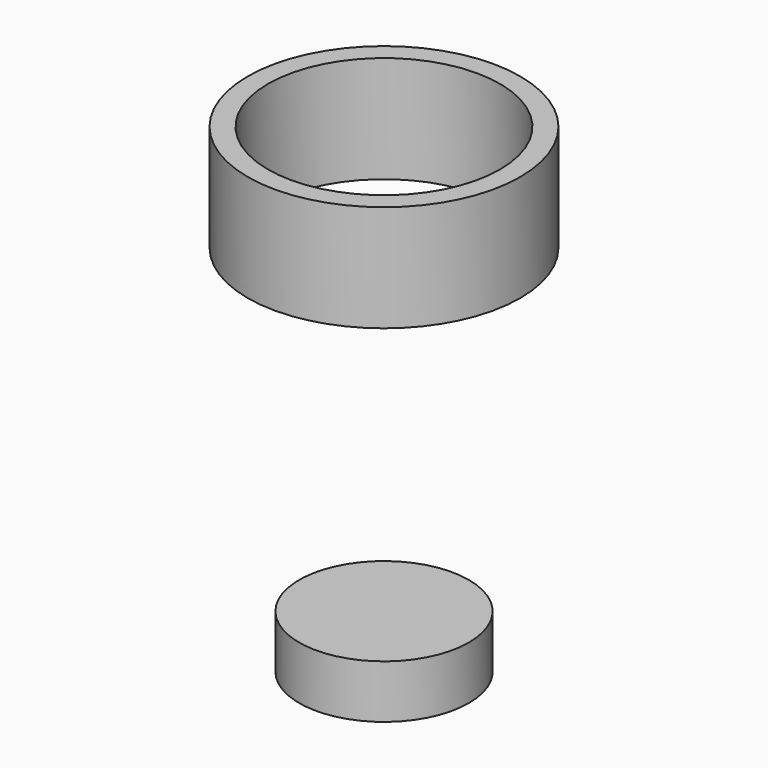
from build123d import *

# Parameters (mm, degrees)
F0_R     = 20.2057
F1_DEPTH = 12.7
F3_R     = 32.4485
F4_DEPTH = 25.4
F6_R     = 27.6183785492
F7_DEPTH = 25.4


# Not quite as in the source:
# - the program builds the solid bodies; features that only make, move or delete a surface that nothing else refers to are left out


with BuildPart() as f1:
    # F0 (on Top) → F1 (new body)
    with BuildSketch(Plane.XY):
        Circle(F0_R)
    extrude(amount=F1_DEPTH)


with BuildPart() as f4:
    # F3 (on offset) → F4 (new body)
    with BuildSketch(Plane.XY.offset(88.9)):
        Circle(F3_R)
    extrude(amount=F4_DEPTH)

    # F6 (on face) → F7 (cut)
    with BuildSketch(Plane.XY.offset(114.3)):
        Circle(F6_R)
    extrude(amount=-F7_DEPTH, mode=Mode.SUBTRACT)


solid = Compound([f1.part, f4.part])
